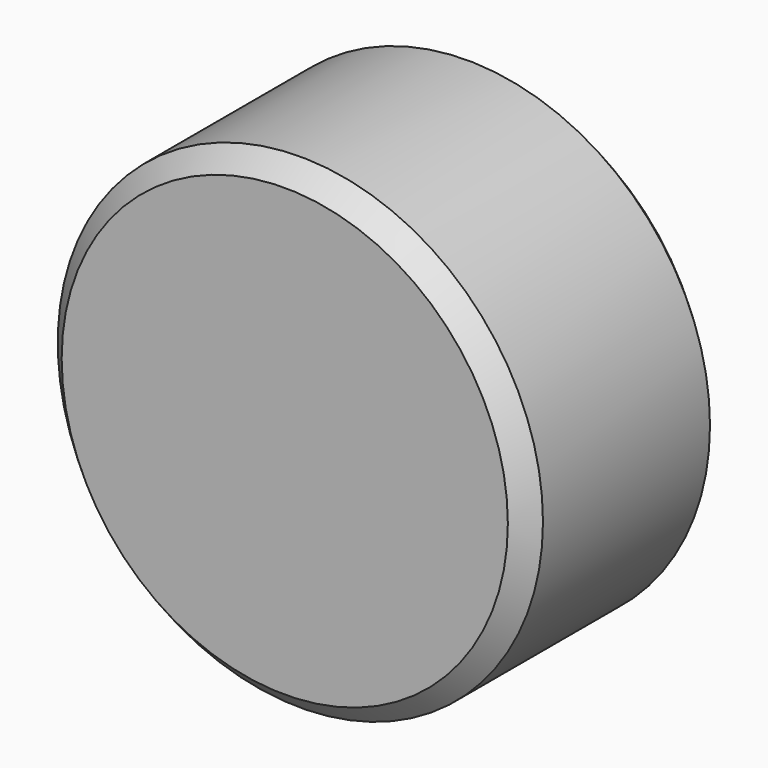
from build123d import *

# Parameters (mm, degrees)
F0_R     = 12.4344228223
F1_DEPTH = 12.7
F2_SIZE  = 1
F3_T     = -1.5


# Not quite as in the source:
# - a fillet or chamfer that OpenCascade refuses, or shapes differently, is made with other operations: its cross-section is extruded or revolved along the edge and cut away or added
# - the program builds the solid bodies; features that only make, move or delete a surface that nothing else refers to are left out


with BuildPart() as f1:
    # F0 (on Front) → F1 (new body)
    with BuildSketch(Plane.XZ):
        Circle(F0_R)
    extrude(amount=F1_DEPTH)

    # F2
    f2_edges = [f1.edges().sort_by_distance(p)[0] for p in [
        (-12.434423, 0, 0),
        (12.434423, -6.35, 0),
        (-12.434423, -12.7, 0),
    ]]
    chamfer(f2_edges, length=F2_SIZE)

    # F3
    f3_openings = [f1.faces().sort_by_distance(p)[0] for p in [
        (0, 0, 0),
    ]]
    offset(amount=F3_T, openings=f3_openings)

    # F5: chamfer of 0.2 on 2 edges, made by hand

    # F5_s1 → F5_t2 (revolve, cut)
    with BuildSketch(Plane.XY):
        Polygon((9.5131024788, 0), (9.454523835, -0.1414213562), (9.3131024788, 0), align=None)
    revolve(axis=Axis((0, 0, 0), (0, 1, 0)), mode=Mode.SUBTRACT)


solid = f1.part
